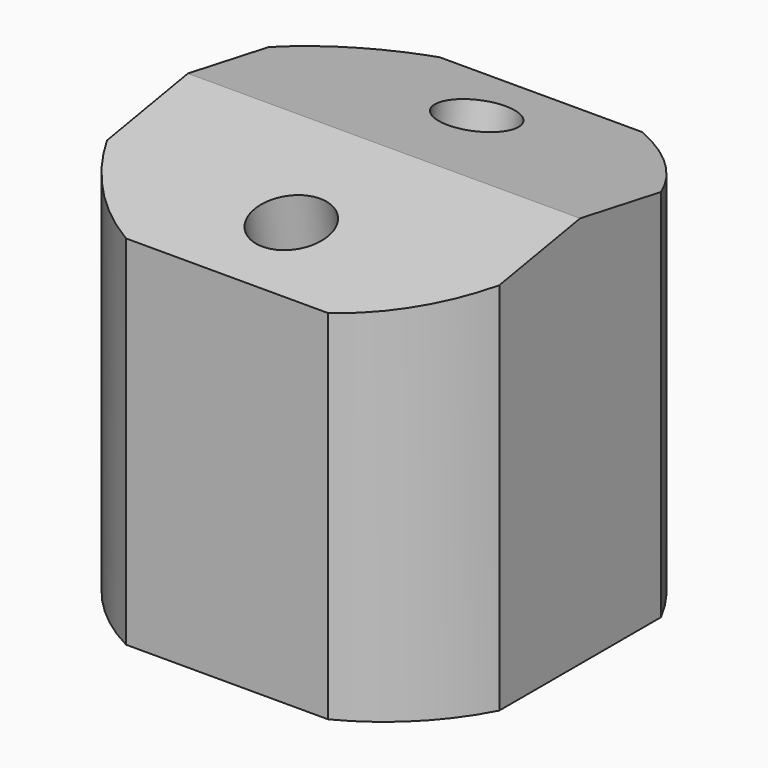
from build123d import *

# Parameters (mm, degrees)
F0_W     = 101.6
F0_H     = 101.6
F1_DEPTH = 50.8
F2_R     = 38.1
F3_DEPTH = 76.2
F5_DEPTH = 50.8
F6_R     = 9.525
F7_DEPTH = 25.4
F9_DEPTH = 127


# Not quite as in the source:
# - a pattern or mirror of a feature is missing from the dataset's text; its kind, count and spacing are read off the source's solid


with BuildPart() as f1:
    # F0 (on Top) → F1 (new body, symmetric)
    with BuildSketch(Plane.XY):
        Rectangle(F0_W, F0_H)
    extrude(amount=F1_DEPTH, both=True)

    # F2 (on face) → F3 (cut)
    with BuildSketch(Plane(origin=(0, 0, -50.8), x_dir=(1, 0, 0), z_dir=(0, 0, -1))):
        Circle(F2_R)
    extrude(amount=-F3_DEPTH, mode=Mode.SUBTRACT)

    # F4 (on Right) → F5 (cut, symmetric)
    with BuildSketch(Plane.YZ):
        Polygon((-50.8, 41.84258938), (0, 50.8), (-50.8, 50.8), align=None)
    f5 = extrude(amount=F5_DEPTH, both=True, mode=Mode.SUBTRACT)

    # F5_copies: F5 across plane
    add(f5.mirror(Plane.ZX), mode=Mode.SUBTRACT)

    # F6 (on face) → F7 (cut)
    with BuildSketch(Plane(origin=(0, -8.6873116405, 49.268192568), x_dir=(1, 0, 0), z_dir=(0, -0.1736481777, 0.984807753))):
        with Locations((0, -21.6586725745)):
            Circle(F6_R)
    f7 = extrude(amount=-F7_DEPTH, mode=Mode.SUBTRACT)

    # F7_copies: F7 across plane
    add(f7.mirror(Plane.ZX.offset(5e-06)), mode=Mode.SUBTRACT)

    # F8 (on face) → F9 (cut)
    with BuildSketch(Plane(origin=(0, 0, -50.8), x_dir=(1, 0, 0), z_dir=(0, 0, -1))):
        with BuildLine():
            ThreePointArc((26.1817207227, 50.8), (40.4111525448, 40.4111525448), (50.8, 26.1817207227))
            Line((50.8, 26.1817207227), (50.8, 50.8))
            Line((50.8, 50.8), (26.1817207227, 50.8))
        make_face()
        with BuildLine():
            Line((50.8, -50.8), (50.8, -26.1817207227))
            ThreePointArc((50.8, -26.1817207227), (40.4111525448, -40.4111525448), (26.1817207227, -50.8))
            Line((26.1817207227, -50.8), (50.8, -50.8))
        make_face()
        with BuildLine():
            Line((-26.1817207227, 50.8), (26.1817207227, 50.8))
            ThreePointArc((26.1817207227, 50.8), (0, 57.15), (-26.1817207227, 50.8))
        make_face()
        with BuildLine():
            ThreePointArc((-50.8, 26.1817207227), (-40.4111525448, 40.4111525448), (-26.1817207227, 50.8))
            Line((-26.1817207227, 50.8), (-50.8, 50.8))
            Line((-50.8, 50.8), (-50.8, 26.1817207227))
        make_face()
        with BuildLine():
            Line((-50.8, -50.8), (-26.1817207227, -50.8))
            ThreePointArc((-26.1817207227, -50.8), (-40.4111525448, -40.4111525448), (-50.8, -26.1817207227))
            Line((-50.8, -26.1817207227), (-50.8, -50.8))
        make_face()
    extrude(amount=-F9_DEPTH, mode=Mode.SUBTRACT)


solid = f1.part
